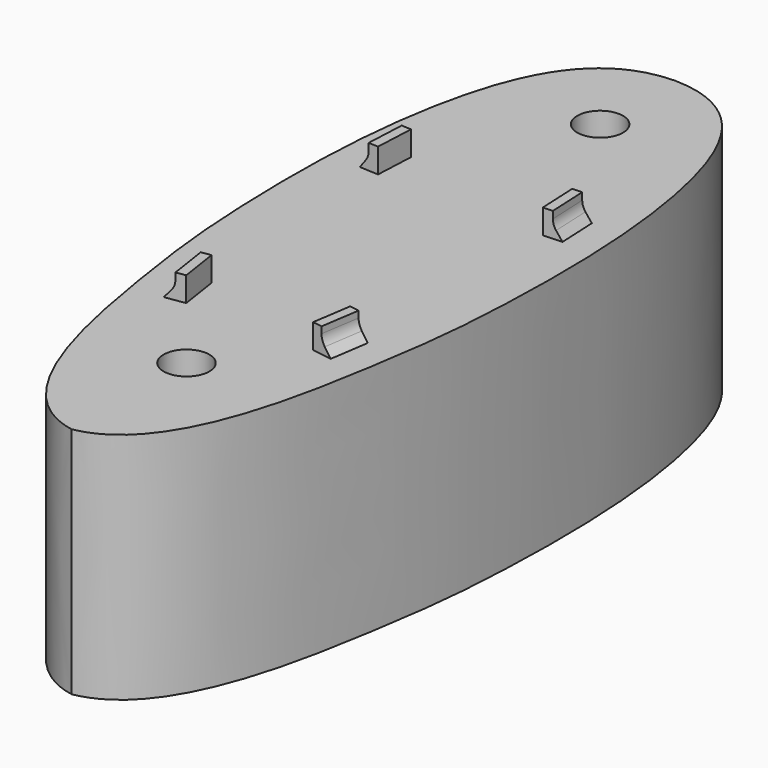
from build123d import *

# Parameters (mm, degrees)
F1_R      = 3.735
F2_DEPTH  = 38.1
F4_DEPTH  = 4
F6_DEPTH  = 6.44
F8_DEPTH  = 6.3670715404
F10_DEPTH = 6.3670715404
F12_DEPTH = 6.44
F13_R     = 2.5
F14_DEPTH = 7


# Not quite as in the source:
# - a feature names something its author has since deleted; it is built from what else it names


with BuildPart() as f2:
    # F1 (on Top) → F2 (new body)
    with BuildSketch(Plane.XY):
        with BuildLine():
            add(Edge.make_bspline(
                [(0, 61.62), (11.5485272162, 61.4039385019), (22.0841192578, 39.7713639929), (22.0172478155, -1.3215032222), (19.7727052767, -22.1995102033), (12.6960353016, -59.3664700438), (0, -61.62)],
                knots=[0, 0, 0, 0, 0.2315513491, 0.5055689387, 0.7231235988, 1, 1, 1, 1], degree=3))
            add(Edge.make_bspline(
                [(0, 61.62), (-11.5485272162, 61.4039385019), (-22.0841192578, 39.7713639929), (-22.0172478155, -1.3215032222), (-19.7727052767, -22.1995102033), (-12.6960353016, -59.3664700438), (0, -61.62)],
                knots=[0, 0, 0, 0, 0.2315513491, 0.5055689387, 0.7231235988, 1, 1, 1, 1], degree=3))
        make_face()
        Polygon((-14.3142142012, -26.7031931663), (-15.512723518, -18.7530249028), (-10.6481931396, -18.0196838229), (-9.4496838229, -25.9698520863), align=None, mode=Mode.SUBTRACT)
        with Locations((0, -38.185)):
            Circle(F1_R, mode=Mode.SUBTRACT)
        Polygon((9.4496838229, -25.9698520863), (10.6481931396, -18.0196838229), (15.512723518, -18.7530249028), (14.3142142012, -26.7031931663), align=None, mode=Mode.SUBTRACT)
        Polygon((-17.3883624322, 17.1146464619), (-17.0129745562, 25.0728694338), (-12.318194576, 24.851417548), (-12.693582452, 16.893194576), align=None, mode=Mode.SUBTRACT)
        Polygon((17.3883624322, 17.1146464619), (12.693582452, 16.893194576), (12.318194576, 24.851417548), (17.0129745562, 25.0728694338), align=None, mode=Mode.SUBTRACT)
        with Locations((0, 46.255)):
            Circle(F1_R, mode=Mode.SUBTRACT)
        Polygon((15.512723518, -18.7530249028), (10.6481931396, -18.0196838229), (9.4496838229, -25.9698520863), (14.3142142012, -26.7031931663), align=None)
        Polygon((10.36, -25.298045226), (11.32, -18.93), (14.6024073408, -19.4248317632), (13.6424073408, -25.7928769892), align=None, mode=Mode.SUBTRACT)
        Polygon((-10.6481931396, -18.0196838229), (-15.512723518, -18.7530249028), (-14.3142142012, -26.7031931663), (-9.4496838229, -25.9698520863), align=None)
        Polygon((-14.6024073408, -19.4248317632), (-11.32, -18.93), (-10.36, -25.298045226), (-13.6424073408, -25.7928769892), align=None, mode=Mode.SUBTRACT)
        Polygon((-12.318194576, 24.851417548), (-17.0129745562, 25.0728694338), (-17.3883624322, 17.1146464619), (-12.693582452, 16.893194576), align=None)
        Polygon((-13.155, 24.09), (-13.455, 17.73), (-16.5515570082, 17.8760640098), (-16.2515570082, 24.2360640098), align=None, mode=Mode.SUBTRACT)
        Polygon((12.318194576, 24.851417548), (12.693582452, 16.893194576), (17.3883624322, 17.1146464619), (17.0129745562, 25.0728694338), align=None)
        Polygon((16.5515570082, 17.8760640098), (13.455, 17.73), (13.155, 24.09), (16.2515570082, 24.2360640098), align=None, mode=Mode.SUBTRACT)
        Polygon((14.6024073408, -19.4248317632), (11.32, -18.93), (10.36, -25.298045226), (13.6424073408, -25.7928769892), align=None)
        Polygon((-10.36, -25.298045226), (-11.32, -18.93), (-14.6024073408, -19.4248317632), (-13.6424073408, -25.7928769892), align=None)
        Polygon((-16.5515570082, 17.8760640098), (-13.455, 17.73), (-13.155, 24.09), (-16.2515570082, 24.2360640098), align=None)
        Polygon((13.155, 24.09), (13.455, 17.73), (16.5515570082, 17.8760640098), (16.2515570082, 24.2360640098), align=None)
    extrude(amount=F2_DEPTH)

    # F3 (on face) → F4 (join)
    with BuildSketch(Plane.XY.offset(38.1)):
        Polygon((-10.36, -25.298045226), (-11.32, -18.93), (-14.6024073408, -19.4248317632), (-13.6424073408, -25.7928769892), align=None)
        Polygon((14.6024073408, -19.4248317632), (11.32, -18.93), (10.36, -25.298045226), (13.6424073408, -25.7928769892), align=None)
        Polygon((13.155, 24.09), (13.455, 17.73), (16.5515570082, 17.8760640098), (16.2515570082, 24.2360640098), align=None)
        Polygon((-16.5515570082, 17.8760640098), (-13.455, 17.73), (-13.155, 24.09), (-16.2515570082, 24.2360640098), align=None)
    extrude(amount=F4_DEPTH)

    # F5 (on face) → F6 (cut, through all)
    with BuildSketch(Plane(origin=(3.4987885373, -23.2087954603, 0), x_dir=(0.9888268984, 0.149068323, 0), z_dir=(0.149068323, -0.9888268984, 0))):
        Polygon((-17.3348802558, 42.1), (-17.3348802558, 38.1), (-15.6033838444, 40.1), (-15.6033838444, 42.1), align=None)
    extrude(amount=-F6_DEPTH, mode=Mode.SUBTRACT)

    # F7 (on face) → F8 (cut, through all)
    with BuildSketch(Plane(origin=(0.8045932866, 17.0573776752, 0), x_dir=(0.9988893575, -0.0471174225, 0), z_dir=(-0.0471174225, -0.9988893575, 0))):
        Polygon((-15.8629482063, 40.1), (-15.8629482063, 42.1), (-17.3754482063, 42.1), (-17.3754482063, 38.1), align=None)
    extrude(amount=-F8_DEPTH, mode=Mode.SUBTRACT)

    # F9 (on face) → F10 (cut, through all)
    with BuildSketch(Plane(origin=(-0.8045932866, 17.0573776752, 0), x_dir=(0.9988893575, 0.0471174225, 0), z_dir=(0.0471174225, -0.9988893575, 0))):
        Polygon((15.8629482063, 42.1), (15.8629482063, 40.1), (17.3754482063, 38.1), (17.3754482063, 42.1), align=None)
    extrude(amount=-F10_DEPTH, mode=Mode.SUBTRACT)

    # F11 (on face) → F12 (cut, through all)
    with BuildSketch(Plane(origin=(-3.4987885373, -23.2087954603, 0), x_dir=(0.9888268984, -0.149068323, 0), z_dir=(-0.149068323, -0.9888268984, 0))):
        Polygon((17.3348802558, 42.1), (15.6028838444, 42.1), (15.6028838444, 40.1), (17.3348802558, 38.1), align=None)
    extrude(amount=-F12_DEPTH, mode=Mode.SUBTRACT)

    # F13
    f13_edges = [f2.edges().sort_by_distance(p)[0] for p in [
        (12.409763, -22.350669, 40.1),
        (14.890737, 20.984799, 40.1),
        (-14.890737, 20.984799, 40.1),
        (-12.410257, -22.350743, 40.1),
    ]]
    fillet(f13_edges, radius=F13_R)

    # F1 (on Top) → F14 (cut)
    with BuildSketch(Plane.XY):
        Polygon((15.512723518, -18.7530249028), (10.6481931396, -18.0196838229), (9.4496838229, -25.9698520863), (14.3142142012, -26.7031931663), align=None)
        Polygon((10.36, -25.298045226), (11.32, -18.93), (14.6024073408, -19.4248317632), (13.6424073408, -25.7928769892), align=None, mode=Mode.SUBTRACT)
        Polygon((-10.6481931396, -18.0196838229), (-15.512723518, -18.7530249028), (-14.3142142012, -26.7031931663), (-9.4496838229, -25.9698520863), align=None)
        Polygon((-14.6024073408, -19.4248317632), (-11.32, -18.93), (-10.36, -25.298045226), (-13.6424073408, -25.7928769892), align=None, mode=Mode.SUBTRACT)
        Polygon((12.318194576, 24.851417548), (12.693582452, 16.893194576), (17.3883624322, 17.1146464619), (17.0129745562, 25.0728694338), align=None)
        Polygon((16.5515570082, 17.8760640098), (13.455, 17.73), (13.155, 24.09), (16.2515570082, 24.2360640098), align=None, mode=Mode.SUBTRACT)
        Polygon((-12.318194576, 24.851417548), (-17.0129745562, 25.0728694338), (-17.3883624322, 17.1146464619), (-12.693582452, 16.893194576), align=None)
        Polygon((-13.155, 24.09), (-13.455, 17.73), (-16.5515570082, 17.8760640098), (-16.2515570082, 24.2360640098), align=None, mode=Mode.SUBTRACT)
        Polygon((-10.36, -25.298045226), (-11.32, -18.93), (-14.6024073408, -19.4248317632), (-13.6424073408, -25.7928769892), align=None)
        Polygon((14.6024073408, -19.4248317632), (11.32, -18.93), (10.36, -25.298045226), (13.6424073408, -25.7928769892), align=None)
        Polygon((13.155, 24.09), (13.455, 17.73), (16.5515570082, 17.8760640098), (16.2515570082, 24.2360640098), align=None)
        Polygon((-16.5515570082, 17.8760640098), (-13.455, 17.73), (-13.155, 24.09), (-16.2515570082, 24.2360640098), align=None)
    extrude(amount=F14_DEPTH, mode=Mode.SUBTRACT)


solid = f2.part
